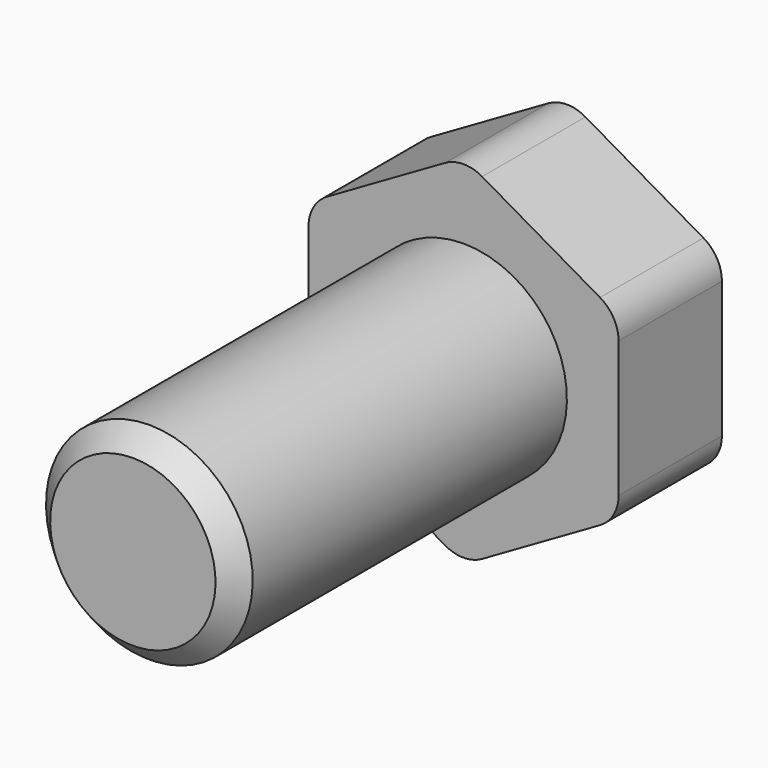
from build123d import *

# Parameters (mm, degrees)
F2_R     = 25.1475
F3_DEPTH = 25


# Not quite as in the source:
# - a feature names something its author has since deleted; it is built from what else it names


with BuildPart() as f1:
    # F0 (on Right) → F1 (revolve)
    with BuildSketch(Plane.YZ):
        Polygon((0, 25.1475), (0, 10), (-38, 10), (-40, 8), (-40, 0), (12.5, 0), (12.5, 25.1475), align=None)
    revolve(axis=Axis((0, -13.75, 0), (0, -1, 0)))

    # F2 (on face) → F3 (cut)
    with BuildSketch(Plane(origin=(0, 12.5, 0), x_dir=(-1, 0, 0), z_dir=(0, 1, 0))):
        Circle(F2_R)
        with BuildLine():
            ThreePointArc((1.7954303246, -16.2839158944), (0, -16.765), (-1.7954303246, -16.2839158944))
            Line((-1.7954303246, -16.2839158944), (-13.2045696754, -9.6968462191))
            ThreePointArc((-13.2045696754, -9.6968462191), (-14.5189158944, -8.3825), (-15, -6.5870696754))
            Line((-15, -6.5870696754), (-15, 6.5870696754))
            ThreePointArc((-15, 6.5870696754), (-14.5189158944, 8.3825), (-13.2045696754, 9.6968462191))
            Line((-13.2045696754, 9.6968462191), (-1.7954303246, 16.2839158944))
            ThreePointArc((-1.7954303246, 16.2839158944), (0, 16.765), (1.7954303246, 16.2839158944))
            Line((1.7954303246, 16.2839158944), (13.2045696754, 9.6968462191))
            ThreePointArc((13.2045696754, 9.6968462191), (14.5189158944, 8.3825), (15, 6.5870696754))
            Line((15, 6.5870696754), (15, -6.5870696754))
            ThreePointArc((15, -6.5870696754), (14.5189158944, -8.3825), (13.2045696754, -9.6968462191))
            Line((13.2045696754, -9.6968462191), (1.7954303246, -16.2839158944))
        make_face(mode=Mode.SUBTRACT)
    extrude(amount=-F3_DEPTH, mode=Mode.SUBTRACT)


solid = f1.part
